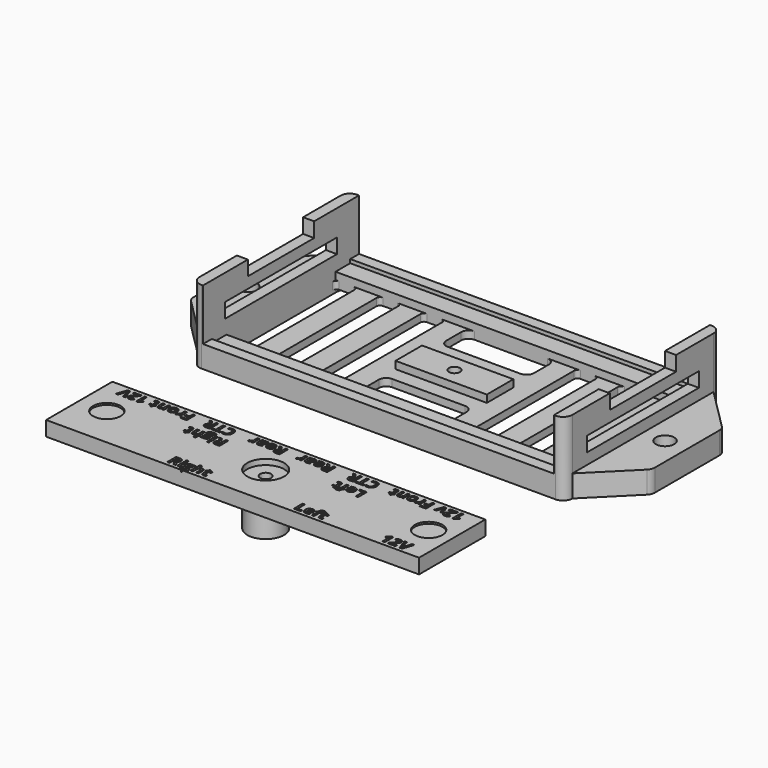
from build123d import *

# Parameters (mm, degrees)
F0_W            = 24.8000000916
F0_H            = 9
F0_W_2          = 95.3
F0_H_2          = 5
F0_R            = 2.5
F0_H_3          = 3
F0_W_3          = 47.65
F0_R_2          = 1.5
F1_DEPTH        = 3
F2_DEPTH        = 17
F3_DEPTH        = 2
F4_DEPTH        = 3
F5_W            = 3
F5_H            = 22.5
F6_W            = 3
F6_H            = 22.5
F7_DEPTH        = 4
F0_W_4          = 101.3
F0_H_4          = 22.5
F0_R_3          = 5
F8_DEPTH        = 4
F9_DEPTH        = 10
F10_DEPTH       = 3
F11_R           = 5
F11_R_2         = 1.5
F12_DEPTH       = 1.5
F13_R           = 6
F13_R_2         = 5
F14_DEPTH       = 1.5
F15_TEXT_SIZE   = 4.254734022
F15_TEXT_SIZE_2 = 4.1666666667
F15_TEXT_SIZE_3 = 4.0404040404
F15_W           = 0.6204427083
F15_H           = 2.2747395833
F15_R           = 3.75
F16_DEPTH       = 0.5
F17_R           = 1.5
F18_DEPTH       = 1
F19_W           = 96.2200004339
F19_H           = 17.4200004339
F19_R           = 7.9304002091
F20_DEPTH       = 2
F22_DEPTH       = 2
F24_W           = 38
F24_H           = 4
F23_W           = 38
F23_H           = 4
F25_DEPTH       = 5.5
F21_R           = 4.5
F21_R_2         = 1.5
F26_DEPTH       = 1


# Not quite as in the source:
# - a feature names something its author has since deleted; it is built from what else it names
# - Text() gives the source's letters only with a copy of the font that has no kerning and outlines rounded to 1/6400 em; it was checked with that copy


with BuildPart() as f1:
    # F0 (on Top) → F1 (new body)
    with BuildSketch(Plane.XY):
        Polygon((49.3014014482, 10.8854821861), (-45.9985985518, 10.8854821861), (-45.9985985518, -26.1145178139), (1.6514014482, -26.1145178139), (49.3014014482, -26.1145178139), align=None)
        with Locations((1.9014014941, -8.6145178139)):
            Rectangle(F0_W, F0_H, mode=Mode.SUBTRACT)
        with Locations((1.6514014482, 13.3854821861)):
            Rectangle(F0_W_2, F0_H_2)
        with BuildLine():
            Line((-48.9985985518, -31.5745178139), (-48.9985985518, 16.3454821861))
            Line((-48.9985985518, 16.3454821861), (-60.2531511942, 5.1096871314))
            ThreePointArc((-60.2531511942, 5.1096871314), (-60.804847016, 4.2851329962), (-60.9985985518, 3.3121385747))
            Line((-60.9985985518, 3.3121385747), (-60.9985985518, -18.5411742026))
            ThreePointArc((-60.9985985518, -18.5411742026), (-60.804847016, -19.514168624), (-60.2531511942, -20.3387227592))
            Line((-60.2531511942, -20.3387227592), (-48.9985985518, -31.5745178139))
        make_face()
        with Locations((-54.9985985518, -7.6145178139)):
            Circle(F0_R, mode=Mode.SUBTRACT)
        with BuildLine():
            Line((63.5559540907, 5.1096871314), (52.3014014482, 16.3454821861))
            Line((52.3014014482, 16.3454821861), (52.3014014482, -31.5745178139))
            Line((52.3014014482, -31.5745178139), (63.5559540907, -20.3387227592))
            ThreePointArc((63.5559540907, -20.3387227592), (64.1076499125, -19.514168624), (64.3014014482, -18.5411742026))
            Line((64.3014014482, -18.5411742026), (64.3014014482, -7.6145178139))
            Line((64.3014014482, -7.6145178139), (64.3014014482, 3.3121385747))
            ThreePointArc((64.3014014482, 3.3121385747), (64.1076499125, 4.2851329962), (63.5559540907, 5.1096871314))
        make_face()
        with Locations((58.3014014482, -7.6145178139)):
            Circle(F0_R, mode=Mode.SUBTRACT)
        with Locations((1.6514014482, 17.3854821861)):
            Rectangle(F0_W_2, F0_H_3)
        Polygon((1.6514014482, -31.1145178139), (-45.9985985518, -31.1145178139), (-45.9985985518, -34.1145178139), (49.3014014482, -34.1145178139), (49.3014014482, -31.1145178139), align=None)
        with Locations((-22.1735985518, -28.6145178139)):
            Rectangle(F0_W_3, F0_H_2)
        with Locations((25.4764014482, -28.6145178139)):
            Rectangle(F0_W_3, F0_H_2)
        with Locations((1.9014014941, -8.6145178139)):
            Rectangle(F0_W, F0_H)
        with Locations((1.9014014941, -8.6145178139)):
            Circle(F0_R_2, mode=Mode.SUBTRACT)
        with BuildLine():
            Line((49.3014014482, 18.8854821861), (49.3014014482, 15.8854821861))
            Line((49.3014014482, 15.8854821861), (49.3014014482, 10.8854821861))
            Line((49.3014014482, 10.8854821861), (49.3014014482, -26.1145178139))
            Line((49.3014014482, -26.1145178139), (49.3014014482, -31.1145178139))
            Line((49.3014014482, -31.1145178139), (49.3014014482, -34.1145178139))
            Line((49.3014014482, -34.1145178139), (49.7614014482, -34.1145178139))
            ThreePointArc((49.7614014482, -34.1145178139), (51.5574526725, -33.3705690381), (52.3014014482, -31.5745178139))
            Line((52.3014014482, -31.5745178139), (52.3014014482, 16.3454821861))
            ThreePointArc((52.3014014482, 16.3454821861), (51.5574526725, 18.1415334103), (49.7614014482, 18.8854821861))
            Line((49.7614014482, 18.8854821861), (49.3014014482, 18.8854821861))
        make_face()
        with BuildLine():
            Line((-45.9985985518, 10.8854821861), (-45.9985985518, 15.8854821861))
            Line((-45.9985985518, 15.8854821861), (-45.9985985518, 18.8854821861))
            Line((-45.9985985518, 18.8854821861), (-46.4585985518, 18.8854821861))
            ThreePointArc((-46.4585985518, 18.8854821861), (-48.254649776, 18.1415334103), (-48.9985985518, 16.3454821861))
            Line((-48.9985985518, 16.3454821861), (-48.9985985518, -31.5745178139))
            ThreePointArc((-48.9985985518, -31.5745178139), (-48.254649776, -33.3705690381), (-46.4585985518, -34.1145178139))
            Line((-46.4585985518, -34.1145178139), (-45.9985985518, -34.1145178139))
            Line((-45.9985985518, -34.1145178139), (-45.9985985518, -31.1145178139))
            Line((-45.9985985518, -31.1145178139), (-45.9985985518, -26.1145178139))
            Line((-45.9985985518, -26.1145178139), (-45.9985985518, 10.8854821861))
        make_face()
    extrude(amount=-F1_DEPTH)

    # F0 (on Top) → F2 (join)
    with BuildSketch(Plane.XY):
        with BuildLine():
            Line((49.3014014482, 18.8854821861), (49.3014014482, 15.8854821861))
            Line((49.3014014482, 15.8854821861), (49.3014014482, 10.8854821861))
            Line((49.3014014482, 10.8854821861), (49.3014014482, -26.1145178139))
            Line((49.3014014482, -26.1145178139), (49.3014014482, -31.1145178139))
            Line((49.3014014482, -31.1145178139), (49.3014014482, -34.1145178139))
            Line((49.3014014482, -34.1145178139), (49.7614014482, -34.1145178139))
            ThreePointArc((49.7614014482, -34.1145178139), (51.5574526725, -33.3705690381), (52.3014014482, -31.5745178139))
            Line((52.3014014482, -31.5745178139), (52.3014014482, 16.3454821861))
            ThreePointArc((52.3014014482, 16.3454821861), (51.5574526725, 18.1415334103), (49.7614014482, 18.8854821861))
            Line((49.7614014482, 18.8854821861), (49.3014014482, 18.8854821861))
        make_face()
        with BuildLine():
            Line((-45.9985985518, 10.8854821861), (-45.9985985518, 15.8854821861))
            Line((-45.9985985518, 15.8854821861), (-45.9985985518, 18.8854821861))
            Line((-45.9985985518, 18.8854821861), (-46.4585985518, 18.8854821861))
            ThreePointArc((-46.4585985518, 18.8854821861), (-48.254649776, 18.1415334103), (-48.9985985518, 16.3454821861))
            Line((-48.9985985518, 16.3454821861), (-48.9985985518, -31.5745178139))
            ThreePointArc((-48.9985985518, -31.5745178139), (-48.254649776, -33.3705690381), (-46.4585985518, -34.1145178139))
            Line((-46.4585985518, -34.1145178139), (-45.9985985518, -34.1145178139))
            Line((-45.9985985518, -34.1145178139), (-45.9985985518, -31.1145178139))
            Line((-45.9985985518, -31.1145178139), (-45.9985985518, -26.1145178139))
            Line((-45.9985985518, -26.1145178139), (-45.9985985518, 10.8854821861))
        make_face()
    extrude(amount=F2_DEPTH)

    # F0 (on Top) → F3 (join)
    with BuildSketch(Plane.XY):
        with Locations((1.9014014941, -8.6145178139)):
            Rectangle(F0_W, F0_H)
        with Locations((1.9014014941, -8.6145178139)):
            Circle(F0_R_2, mode=Mode.SUBTRACT)
        with Locations((1.6514014482, 13.3854821861)):
            Rectangle(F0_W_2, F0_H_2)
        with Locations((-22.1735985518, -28.6145178139)):
            Rectangle(F0_W_3, F0_H_2)
        with Locations((25.4764014482, -28.6145178139)):
            Rectangle(F0_W_3, F0_H_2)
    extrude(amount=F3_DEPTH)

    # F0 (on Top) → F4 (join)
    with BuildSketch(Plane.XY):
        with Locations((1.6514014482, 17.3854821861)):
            Rectangle(F0_W_2, F0_H_3)
        Polygon((1.6514014482, -31.1145178139), (-45.9985985518, -31.1145178139), (-45.9985985518, -34.1145178139), (49.3014014482, -34.1145178139), (49.3014014482, -31.1145178139), align=None)
    extrude(amount=F4_DEPTH)

    # F5 (on face) + F6 (on face) → F7 (cut)
    with BuildSketch(Plane.XY.offset(17)):
        with Locations((50.8014014482, -7.6145178139)):
            Rectangle(F5_W, F5_H)
    with BuildSketch(Plane.XY.offset(17)):
        with Locations((-47.4985985518, -7.6145178139)):
            Rectangle(F6_W, F6_H)
    extrude(amount=-F7_DEPTH, mode=Mode.SUBTRACT)

    # F0 (on Top) → F10 (join)
    with BuildSketch(Plane.XY):
        with BuildLine():
            Line((-48.9985985518, -31.5745178139), (-48.9985985518, 16.3454821861))
            Line((-48.9985985518, 16.3454821861), (-60.2531511942, 5.1096871314))
            ThreePointArc((-60.2531511942, 5.1096871314), (-60.804847016, 4.2851329962), (-60.9985985518, 3.3121385747))
            Line((-60.9985985518, 3.3121385747), (-60.9985985518, -18.5411742026))
            ThreePointArc((-60.9985985518, -18.5411742026), (-60.804847016, -19.514168624), (-60.2531511942, -20.3387227592))
            Line((-60.2531511942, -20.3387227592), (-48.9985985518, -31.5745178139))
        make_face()
        with Locations((-54.9985985518, -7.6145178139)):
            Circle(F0_R, mode=Mode.SUBTRACT)
        with BuildLine():
            Line((63.5559540907, 5.1096871314), (52.3014014482, 16.3454821861))
            Line((52.3014014482, 16.3454821861), (52.3014014482, -31.5745178139))
            Line((52.3014014482, -31.5745178139), (63.5559540907, -20.3387227592))
            ThreePointArc((63.5559540907, -20.3387227592), (64.1076499125, -19.514168624), (64.3014014482, -18.5411742026))
            Line((64.3014014482, -18.5411742026), (64.3014014482, -7.6145178139))
            Line((64.3014014482, -7.6145178139), (64.3014014482, 3.3121385747))
            ThreePointArc((64.3014014482, 3.3121385747), (64.1076499125, 4.2851329962), (63.5559540907, 5.1096871314))
        make_face()
        with Locations((58.3014014482, -7.6145178139)):
            Circle(F0_R, mode=Mode.SUBTRACT)
    extrude(amount=F10_DEPTH)

    # F17 (on face) → F18 (cut)
    with BuildSketch(Plane(origin=(0, 0, -3), x_dir=(1, 0, 0), z_dir=(0, 0, -1))):
        with BuildLine():
            ThreePointArc((-45.9985985518, -10.8854821861), (-44.5341324577, -14.421016092), (-40.9985985518, -15.8854821861))
            Line((-40.9985985518, -15.8854821861), (44.3014014482, -15.8854821861))
            ThreePointArc((44.3014014482, -15.8854821861), (47.8369353542, -14.421016092), (49.3014014482, -10.8854821861))
            Line((49.3014014482, -10.8854821861), (49.3014014482, 26.1145178139))
            ThreePointArc((49.3014014482, 26.1145178139), (47.8369353542, 29.6500517199), (44.3014014482, 31.1145178139))
            Line((44.3014014482, 31.1145178139), (-40.9985985518, 31.1145178139))
            ThreePointArc((-40.9985985518, 31.1145178139), (-44.5341324577, 29.6500517199), (-45.9985985518, 26.1145178139))
            Line((-45.9985985518, 26.1145178139), (-45.9985985518, -10.8854821861))
        make_face()
        with Locations((1.9014014941, 8.6145178139)):
            Circle(F17_R, mode=Mode.SUBTRACT)
    extrude(amount=-F18_DEPTH, mode=Mode.SUBTRACT)

    # F21 (on face) → F22 (cut)
    with BuildSketch(Plane(origin=(0, 0, -2), x_dir=(1, 0, 0), z_dir=(0, 0, -1))):
        with BuildLine():
            ThreePointArc((48.3014014482, -10.8854821861), (49.0085082294, -10.5925889673), (49.3014014482, -9.8854821861))
            Line((49.3014014482, -9.8854821861), (49.3014014482, 25.1145178139))
            ThreePointArc((49.3014014482, 25.1145178139), (49.0085082294, 25.8216245951), (48.3014014482, 26.1145178139))
            Line((48.3014014482, 26.1145178139), (44.3451514482, 26.1145178139))
            ThreePointArc((44.3451514482, 26.1145178139), (43.6380446671, 25.8216245951), (43.3451514482, 25.1145178139))
            Line((43.3451514482, 25.1145178139), (43.3451514482, -9.8854821861))
            ThreePointArc((43.3451514482, -9.8854821861), (43.6380446671, -10.5925889673), (44.3451514482, -10.8854821861))
            Line((44.3451514482, -10.8854821861), (48.3014014482, -10.8854821861))
        make_face()
        with BuildLine():
            Line((37.3889014482, -9.8854821861), (37.3889014482, 25.1145178139))
            ThreePointArc((37.3889014482, 25.1145178139), (37.0960082294, 25.8216245951), (36.3889014482, 26.1145178139))
            Line((36.3889014482, 26.1145178139), (32.4326514482, 26.1145178139))
            ThreePointArc((32.4326514482, 26.1145178139), (31.7255446671, 25.8216245951), (31.4326514482, 25.1145178139))
            Line((31.4326514482, 25.1145178139), (31.4326514482, -9.8854821861))
            ThreePointArc((31.4326514482, -9.8854821861), (31.7255446671, -10.5925889673), (32.4326514482, -10.8854821861))
            Line((32.4326514482, -10.8854821861), (36.3889014482, -10.8854821861))
            ThreePointArc((36.3889014482, -10.8854821861), (37.0960082294, -10.5925889673), (37.3889014482, -9.8854821861))
        make_face()
        with BuildLine():
            ThreePointArc((24.4764014482, -10.8854821861), (25.1835082294, -10.5925889673), (25.4764014482, -9.8854821861))
            Line((25.4764014482, -9.8854821861), (25.4764014482, 25.1145178139))
            ThreePointArc((25.4764014482, 25.1145178139), (25.1835082294, 25.8216245951), (24.4764014482, 26.1145178139))
            Line((24.4764014482, 26.1145178139), (20.5201514482, 26.1145178139))
            ThreePointArc((20.5201514482, 26.1145178139), (19.8130446671, 25.8216245951), (19.5201514482, 25.1145178139))
            Line((19.5201514482, 25.1145178139), (19.5201514482, -9.8854821861))
            ThreePointArc((19.5201514482, -9.8854821861), (19.8130446671, -10.5925889673), (20.5201514482, -10.8854821861))
            Line((20.5201514482, -10.8854821861), (24.4764014482, -10.8854821861))
        make_face()
        with BuildLine():
            Line((-22.1735985518, 25.1145178139), (-22.1735985518, -9.8854821861))
            ThreePointArc((-22.1735985518, -9.8854821861), (-21.8807053329, -10.5925889673), (-21.1735985518, -10.8854821861))
            Line((-21.1735985518, -10.8854821861), (-17.2173485518, -10.8854821861))
            ThreePointArc((-17.2173485518, -10.8854821861), (-16.5102417706, -10.5925889673), (-16.2173485518, -9.8854821861))
            Line((-16.2173485518, -9.8854821861), (-16.2173485518, 25.1145178139))
            ThreePointArc((-16.2173485518, 25.1145178139), (-16.5102417706, 25.8216245951), (-17.2173485518, 26.1145178139))
            Line((-17.2173485518, 26.1145178139), (-21.1735985518, 26.1145178139))
            ThreePointArc((-21.1735985518, 26.1145178139), (-21.8807053329, 25.8216245951), (-22.1735985518, 25.1145178139))
        make_face()
        with BuildLine():
            ThreePointArc((-33.0860985518, 26.1145178139), (-33.7932053329, 25.8216245951), (-34.0860985518, 25.1145178139))
            Line((-34.0860985518, 25.1145178139), (-34.0860985518, -9.8854821861))
            ThreePointArc((-34.0860985518, -9.8854821861), (-33.7932053329, -10.5925889673), (-33.0860985518, -10.8854821861))
            Line((-33.0860985518, -10.8854821861), (-29.1298485518, -10.8854821861))
            ThreePointArc((-29.1298485518, -10.8854821861), (-28.4227417706, -10.5925889673), (-28.1298485518, -9.8854821861))
            Line((-28.1298485518, -9.8854821861), (-28.1298485518, 25.1145178139))
            ThreePointArc((-28.1298485518, 25.1145178139), (-28.4227417706, 25.8216245951), (-29.1298485518, 26.1145178139))
            Line((-29.1298485518, 26.1145178139), (-33.0860985518, 26.1145178139))
        make_face()
        with BuildLine():
            ThreePointArc((-45.9985985518, -9.8854821861), (-45.7057053329, -10.5925889673), (-44.9985985518, -10.8854821861))
            Line((-44.9985985518, -10.8854821861), (-41.0423485518, -10.8854821861))
            ThreePointArc((-41.0423485518, -10.8854821861), (-40.3352417706, -10.5925889673), (-40.0423485518, -9.8854821861))
            Line((-40.0423485518, -9.8854821861), (-40.0423485518, 25.1145178139))
            ThreePointArc((-40.0423485518, 25.1145178139), (-40.3352417706, 25.8216245951), (-41.0423485518, 26.1145178139))
            Line((-41.0423485518, 26.1145178139), (-44.9985985518, 26.1145178139))
            ThreePointArc((-44.9985985518, 26.1145178139), (-45.7057053329, 25.8216245951), (-45.9985985518, 25.1145178139))
            Line((-45.9985985518, 25.1145178139), (-45.9985985518, -9.8854821861))
        make_face()
        with BuildLine():
            ThreePointArc((13.5639014482, 24.1145178139), (12.9781150106, 25.5287313763), (11.5639014482, 26.1145178139))
            Line((11.5639014482, 26.1145178139), (-8.2610985518, 26.1145178139))
            ThreePointArc((-8.2610985518, 26.1145178139), (-9.6753121141, 25.5287313763), (-10.2610985518, 24.1145178139))
            Line((-10.2610985518, 24.1145178139), (-10.2610985518, 19.0735178139))
            ThreePointArc((-10.2610985518, 19.0735178139), (-9.6753121141, 17.6593042515), (-8.2610985518, 17.0735178139))
            Line((-8.2610985518, 17.0735178139), (11.5639014482, 17.0735178139))
            ThreePointArc((11.5639014482, 17.0735178139), (12.9781150106, 17.6593042515), (13.5639014482, 19.0735178139))
            Line((13.5639014482, 19.0735178139), (13.5639014482, 24.1145178139))
        make_face()
        with BuildLine():
            Line((-8.2610985518, -10.8854821861), (11.5639014482, -10.8854821861))
            ThreePointArc((11.5639014482, -10.8854821861), (12.9781150106, -10.2996957485), (13.5639014482, -8.8854821861))
            Line((13.5639014482, -8.8854821861), (13.5639014482, -3.8114821861))
            ThreePointArc((13.5639014482, -3.8114821861), (12.9781150106, -2.3972686237), (11.5639014482, -1.8114821861))
            Line((11.5639014482, -1.8114821861), (-8.2610985518, -1.8114821861))
            ThreePointArc((-8.2610985518, -1.8114821861), (-9.6753121141, -2.3972686237), (-10.2610985518, -3.8114821861))
            Line((-10.2610985518, -3.8114821861), (-10.2610985518, -8.8854821861))
            ThreePointArc((-10.2610985518, -8.8854821861), (-9.6753121141, -10.2996957485), (-8.2610985518, -10.8854821861))
        make_face()
    extrude(amount=-F22_DEPTH, mode=Mode.SUBTRACT)

    # F24 (on face) + F23 (on face) → F25 (cut, symmetric)
    with BuildSketch(Plane(origin=(-48.9985985518, 0, 0), x_dir=(0, -1, 0), z_dir=(-1, 0, 0))):
        with Locations((7.6145178139, 8)):
            Rectangle(F24_W, F24_H)
    with BuildSketch(Plane.YZ.offset(52.3014014482)):
        with Locations((-7.6145178139, 8)):
            Rectangle(F23_W, F23_H)
    extrude(amount=F25_DEPTH, both=True, dir=(-1, 0, 0), mode=Mode.SUBTRACT)

    # F21 (on face) → F26 (join, through all)
    with BuildSketch(Plane(origin=(0, 0, -2), x_dir=(1, 0, 0), z_dir=(0, 0, -1))):
        with Locations((1.9014014941, 8.6145178139)):
            Circle(F21_R)
        with Locations((1.9014014941, 8.6145178139)):
            Circle(F21_R_2, mode=Mode.SUBTRACT)
    extrude(amount=F26_DEPTH)


with BuildPart() as f8:
    # F0 (on Top) → F8 (new body)
    with BuildSketch(Plane.XY):
        with Locations((1.6514019907, -72.3777604103)):
            Rectangle(F0_W_4, F0_H_4)
        with Locations((1.6514019907, -72.3777604103)):
            Circle(F0_R_3, mode=Mode.SUBTRACT)
        with Locations((1.6514019907, -72.3777604103)):
            Circle(F0_R_3)
        with Locations((1.6514019907, -72.3777604103)):
            Circle(F0_R_2, mode=Mode.SUBTRACT)
    extrude(amount=F8_DEPTH)

    # F0 (on Top) → F9 (join)
    with BuildSketch(Plane.XY):
        with Locations((1.6514019907, -72.3777604103)):
            Circle(F0_R_3)
        with Locations((1.6514019907, -72.3777604103)):
            Circle(F0_R_2, mode=Mode.SUBTRACT)
    extrude(amount=-F9_DEPTH)

    # F11 (on face) → F12 (cut)
    with BuildSketch(Plane.XY.offset(4)):
        with Locations((1.6514019907, -72.3777604103)):
            Circle(F11_R)
        with Locations((1.6514019907, -72.3777604103)):
            Circle(F11_R_2, mode=Mode.SUBTRACT)
    extrude(amount=-F12_DEPTH, mode=Mode.SUBTRACT)

    # F13 (on face) → F14 (join)
    with BuildSketch(Plane.XY):
        with Locations((1.6514019907, -72.3777604103)):
            Circle(F13_R)
        with Locations((1.6514019907, -72.3777604103)):
            Circle(F13_R_2, mode=Mode.SUBTRACT)
    extrude(amount=-F14_DEPTH)

    # F15 (on face) → F16 (cut)
    with BuildSketch(Plane.XY.offset(4)):
        with Locations(Location((48.2781432374, -62.1277615428), (0, 0, 180))):
            Text('12v', F15_TEXT_SIZE, font='Open Sans', font_style=FontStyle.BOLD, text_align=(TextAlign.LEFT, TextAlign.BOTTOM))
        with Locations(Location((39.7224306365, -62.1277615428), (0, 0, 180))):
            Text('Front', F15_TEXT_SIZE_2, font='Open Sans', font_style=FontStyle.BOLD, text_align=(TextAlign.LEFT, TextAlign.BOTTOM))
        with Locations(Location((25.045672824, -62.1277615428), (0, 0, 180))):
            Text('CTR', F15_TEXT_SIZE_2, font='Open Sans', font_style=FontStyle.BOLD, text_align=(TextAlign.LEFT, TextAlign.BOTTOM))
        with Locations(Location((25.188250949, -67.0007616282), (0, 0, 180))):
            Text('Left', F15_TEXT_SIZE_2, font='Open Sans', font_style=FontStyle.BOLD, text_align=(TextAlign.LEFT, TextAlign.BOTTOM))
        with Locations(Location((12.9034202198, -62.1277638078), (0, 0, 180))):
            Text('Rear', F15_TEXT_SIZE_2, font='Open Sans', font_style=FontStyle.BOLD, text_align=(TextAlign.LEFT, TextAlign.BOTTOM))
        with Locations(Location((-0.0965797802, -62.1277615428), (0, 0, 180))):
            Text('Rear', F15_TEXT_SIZE_2, font='Open Sans', font_style=FontStyle.BOLD, text_align=(TextAlign.LEFT, TextAlign.BOTTOM))
        with Locations(Location((-13.954327176, -62.1277615428), (0, 0, 180))):
            Text('CTR', F15_TEXT_SIZE_2, font='Open Sans', font_style=FontStyle.BOLD, text_align=(TextAlign.LEFT, TextAlign.BOTTOM))
        with Locations(Location((-12.4689761202, -67.0007615428), (0, 0, 180))):
            Text('Right', F15_TEXT_SIZE_2, font='Open Sans', font_style=FontStyle.BOLD, text_align=(TextAlign.LEFT, TextAlign.BOTTOM))
        with Locations(Location((-25.2775693635, -62.1277615428), (0, 0, 180))):
            Text('Front', F15_TEXT_SIZE_2, font='Open Sans', font_style=FontStyle.BOLD, text_align=(TextAlign.LEFT, TextAlign.BOTTOM))
        with Locations(Location((-37.7485980093, -62.1580645731), (0, 0, 180))):
            Text('12V', F15_TEXT_SIZE_3, font='Open Sans', font_style=FontStyle.BOLD, text_align=(TextAlign.LEFT, TextAlign.BOTTOM))
        with BuildLine():
            Line((-16.2230120718, -82.6277583838), (-16.2230120718, -81.4864823421))
            Line((-16.2230120718, -81.4864823421), (-15.8877256135, -81.4864823421))
            Line((-15.8877256135, -81.4864823421), (-15.1774391552, -82.6277583838))
            Line((-15.1774391552, -82.6277583838), (-14.4775693635, -82.6277583838))
            add(Edge.make_bspline(
                [(-15.3525693635, -81.3315344254), (-14.6806943635, -82.3347896338), (-14.4775693635, -82.6277583838)],
                knots=[0, 0, 0, 1, 1, 1], degree=2))
            add(Edge.make_bspline(
                [(-14.943389676, -81.0112219254), (-15.0875954052, -81.2156490088), (-15.3525693635, -81.3315344254)],
                knots=[0, 0, 0, 1, 1, 1], degree=2))
            add(Edge.make_bspline(
                [(-14.7991839468, -80.5444250504), (-14.7991839468, -80.8067948421), (-14.943389676, -81.0112219254)],
                knots=[0, 0, 0, 1, 1, 1], degree=2))
            add(Edge.make_bspline(
                [(-15.089874051, -79.8738521338), (-14.7991839468, -80.0945552588), (-14.7991839468, -80.5444250504)],
                knots=[0, 0, 0, 1, 1, 1], degree=2))
            add(Edge.make_bspline(
                [(-15.9873349885, -79.6531490088), (-15.3805641552, -79.6531490088), (-15.089874051, -79.8738521338)],
                knots=[0, 0, 0, 1, 1, 1], degree=2))
            Line((-15.9873349885, -79.6531490088), (-16.8538714468, -79.6531490088))
            Line((-16.8538714468, -79.6531490088), (-16.8538714468, -82.6277583838))
            Line((-16.8538714468, -82.6277583838), (-16.2230120718, -82.6277583838))
        make_face()
        with BuildLine():
            Line((-16.0198870718, -80.9734615088), (-16.2230120718, -80.9734615088))
            Line((-16.2230120718, -80.9734615088), (-16.2230120718, -80.1700760921))
            Line((-16.2230120718, -80.1700760921), (-16.0316058218, -80.1700760921))
            add(Edge.make_bspline(
                [(-15.5814105093, -80.2595943213), (-15.7269183218, -80.1700760921), (-16.0316058218, -80.1700760921)],
                knots=[0, 0, 0, 1, 1, 1], degree=2))
            add(Edge.make_bspline(
                [(-15.4359026968, -80.5607010921), (-15.4359026968, -80.3491125504), (-15.5814105093, -80.2595943213)],
                knots=[0, 0, 0, 1, 1, 1], degree=2))
            add(Edge.make_bspline(
                [(-15.578155301, -80.8738521338), (-15.4359026968, -80.7742427588), (-15.4359026968, -80.5607010921)],
                knots=[0, 0, 0, 1, 1, 1], degree=2))
            add(Edge.make_bspline(
                [(-16.0198870718, -80.9734615088), (-15.7204079052, -80.9734615088), (-15.578155301, -80.8738521338)],
                knots=[0, 0, 0, 1, 1, 1], degree=2))
        make_face(mode=Mode.SUBTRACT)
        with BuildLine():
            add(Edge.make_bspline(
                [(-14.1787412385, -79.7651281754), (-14.1787412385, -79.4617427588), (-13.8408506135, -79.4617427588)],
                knots=[0, 0, 0, 1, 1, 1], degree=2))
            add(Edge.make_bspline(
                [(-13.8408506135, -80.0704667171), (-14.1787412385, -80.0704667171), (-14.1787412385, -79.7651281754)],
                knots=[0, 0, 0, 1, 1, 1], degree=2))
            add(Edge.make_bspline(
                [(-13.5872698843, -79.9900630713), (-13.6715797802, -80.0704667171), (-13.8408506135, -80.0704667171)],
                knots=[0, 0, 0, 1, 1, 1], degree=2))
            add(Edge.make_bspline(
                [(-13.5029599885, -79.7651281754), (-13.5029599885, -79.9096594254), (-13.5872698843, -79.9900630713)],
                knots=[0, 0, 0, 1, 1, 1], degree=2))
            add(Edge.make_bspline(
                [(-13.8408506135, -79.4617427588), (-13.5029599885, -79.4617427588), (-13.5029599885, -79.7651281754)],
                knots=[0, 0, 0, 1, 1, 1], degree=2))
        make_face()
        with Locations((-13.841827176, -81.4903885921)):
            Rectangle(F15_W, F15_H)
        with BuildLine():
            add(Edge.make_bspline(
                [(-12.2976699022, -83.6277604103), (-12.7133493907, -83.6143693222), (-12.9424131135, -83.4630448421)],
                knots=[0.0884925433, 0.0884925433, 0.0884925433, 1, 1, 1], degree=2))
            Line((-12.2976699022, -83.6277604103), (-12.1211642128, -83.6277604103))
            add(Edge.make_bspline(
                [(-11.6985980093, -83.5814627277), (-11.8880167396, -83.6211940979), (-12.1211642128, -83.6277604103)],
                knots=[0.5345726688, 0.5345726688, 0.5345726688, 0.9230798932, 0.9230798932, 0.9230798932], degree=2))
            add(Edge.make_bspline(
                [(-11.2601214468, -83.4093339046), (-11.4379643074, -83.5267937195), (-11.6985980093, -83.5814627277)],
                knots=[0, 0, 0, 0.5345726688, 0.5345726688, 0.5345726688], degree=2))
            add(Edge.make_bspline(
                [(-10.9274391552, -82.7905188004), (-10.9274391552, -83.1896073421), (-11.2601214468, -83.4093339046)],
                knots=[0, 0, 0, 1, 1, 1], degree=2))
            add(Edge.make_bspline(
                [(-11.1237282177, -82.3185135921), (-10.9274391552, -82.4793208838), (-10.9274391552, -82.7905188004)],
                knots=[0, 0, 0, 1, 1, 1], degree=2))
            add(Edge.make_bspline(
                [(-11.6943662385, -82.1577063004), (-11.3200172802, -82.1577063004), (-11.1237282177, -82.3185135921)],
                knots=[0, 0, 0, 1, 1, 1], degree=2))
            Line((-11.6943662385, -82.1577063004), (-12.0810849885, -82.1577063004))
            add(Edge.make_bspline(
                [(-12.4228818635, -82.0235917171), (-12.4228818635, -82.1577063004), (-12.0810849885, -82.1577063004)],
                knots=[0, 0, 0, 1, 1, 1], degree=2))
            add(Edge.make_bspline(
                [(-12.3271787385, -81.8608313004), (-12.4228818635, -81.9337479671), (-12.4228818635, -82.0235917171)],
                knots=[0, 0, 0, 1, 1, 1], degree=2))
            Line((-12.3271787385, -81.8608313004), (-12.2353818635, -81.8705969254))
            Line((-12.2353818635, -81.8705969254), (-12.1234026968, -81.8771073421))
            add(Edge.make_bspline(
                [(-11.4147438427, -81.6726802588), (-11.6702776968, -81.8771073421), (-12.1234026968, -81.8771073421)],
                knots=[0, 0, 0, 1, 1, 1], degree=2))
            add(Edge.make_bspline(
                [(-11.1592099885, -81.1017167171), (-11.1592099885, -81.4682531754), (-11.4147438427, -81.6726802588)],
                knots=[0, 0, 0, 1, 1, 1], degree=2))
            add(Edge.make_bspline(
                [(-11.2568662385, -80.7599198421), (-11.1592099885, -80.9129146338), (-11.1592099885, -81.1017167171)],
                knots=[0, 0, 0, 1, 1, 1], degree=2))
            Line((-11.2568662385, -80.7599198421), (-10.9007464468, -80.6687740088))
            Line((-10.9007464468, -80.6687740088), (-10.9007464468, -80.3530188004))
            Line((-10.9007464468, -80.3530188004), (-11.6943662385, -80.3530188004))
            add(Edge.make_bspline(
                [(-11.8620094677, -80.3279536963), (-11.7308245718, -80.3452063004), (-11.6943662385, -80.3530188004)],
                knots=[0, 0, 0, 1, 1, 1], degree=2))
            add(Edge.make_bspline(
                [(-12.0888974885, -80.3107010921), (-11.9931943635, -80.3107010921), (-11.8620094677, -80.3279536963)],
                knots=[0, 0, 0, 1, 1, 1], degree=2))
            add(Edge.make_bspline(
                [(-12.7809547802, -80.5141516129), (-12.5387672802, -80.3107010921), (-12.0888974885, -80.3107010921)],
                knots=[0, 0, 0, 1, 1, 1], degree=2))
            add(Edge.make_bspline(
                [(-13.0231422802, -81.0893469254), (-13.0231422802, -80.7176021338), (-12.7809547802, -80.5141516129)],
                knots=[0, 0, 0, 1, 1, 1], degree=2))
            add(Edge.make_bspline(
                [(-12.9183245718, -81.4926672379), (-13.0231422802, -81.3217688004), (-13.0231422802, -81.0893469254)],
                knots=[0, 0, 0, 1, 1, 1], degree=2))
            add(Edge.make_bspline(
                [(-12.6344704052, -81.7403885921), (-12.8135068635, -81.6635656754), (-12.9183245718, -81.4926672379)],
                knots=[0, 0, 0, 1, 1, 1], degree=2))
            add(Edge.make_bspline(
                [(-12.8522438427, -81.9106359879), (-12.7770485302, -81.8243729671), (-12.6344704052, -81.7403885921)],
                knots=[0, 0, 0, 1, 1, 1], degree=2))
            add(Edge.make_bspline(
                [(-12.9274391552, -82.1271073421), (-12.9274391552, -81.9968990088), (-12.8522438427, -81.9106359879)],
                knots=[0, 0, 0, 1, 1, 1], degree=2))
            add(Edge.make_bspline(
                [(-12.8561500927, -82.3237219254), (-12.9274391552, -82.2312740088), (-12.9274391552, -82.1271073421)],
                knots=[0, 0, 0, 1, 1, 1], degree=2))
            add(Edge.make_bspline(
                [(-12.6891579052, -82.4565344254), (-12.7848610302, -82.4161698421), (-12.8561500927, -82.3237219254)],
                knots=[0, 0, 0, 1, 1, 1], degree=2))
            add(Edge.make_bspline(
                [(-13.0654599885, -82.6541255713), (-12.9372047802, -82.5157792171), (-12.6891579052, -82.4565344254)],
                knots=[0, 0, 0, 1, 1, 1], degree=2))
            add(Edge.make_bspline(
                [(-13.1937151968, -82.9982010921), (-13.1937151968, -82.7924719254), (-13.0654599885, -82.6541255713)],
                knots=[0, 0, 0, 1, 1, 1], degree=2))
            add(Edge.make_bspline(
                [(-12.9424131135, -83.4630448421), (-13.1937151968, -83.2970292171), (-13.1937151968, -82.9982010921)],
                knots=[0, 0, 0, 1, 1, 1], degree=2))
        make_face()
        with BuildLine():
            add(Edge.make_bspline(
                [(-11.6985980093, -83.1469899694), (-11.6818203751, -83.1399721206), (-11.666045926, -83.1323156754)],
                knots=[0.9165936185, 0.9165936185, 0.9165936185, 1, 1, 1], degree=2))
            add(Edge.make_bspline(
                [(-12.1885068635, -83.2241125504), (-11.8829756574, -83.2241125504), (-11.6985980093, -83.1469899694)],
                knots=[0, 0, 0, 0.9165936185, 0.9165936185, 0.9165936185], degree=2))
            add(Edge.make_bspline(
                [(-12.5335589468, -83.1508703629), (-12.4105120718, -83.2241125504), (-12.1885068635, -83.2241125504)],
                knots=[0, 0, 0, 1, 1, 1], degree=2))
            add(Edge.make_bspline(
                [(-12.6566058218, -82.9493729671), (-12.6566058218, -83.0776281754), (-12.5335589468, -83.1508703629)],
                knots=[0, 0, 0, 1, 1, 1], degree=2))
            add(Edge.make_bspline(
                [(-12.5416969677, -82.7368078629), (-12.6566058218, -82.8172115088), (-12.6566058218, -82.9493729671)],
                knots=[0, 0, 0, 1, 1, 1], degree=2))
            add(Edge.make_bspline(
                [(-12.2562151968, -82.6564042171), (-12.4267881135, -82.6564042171), (-12.5416969677, -82.7368078629)],
                knots=[0, 0, 0, 1, 1, 1], degree=2))
            Line((-12.2562151968, -82.6564042171), (-11.9346006135, -82.6564042171))
            add(Edge.make_bspline(
                [(-11.6985980093, -82.6737885249), (-11.7947530313, -82.6564042171), (-11.9346006135, -82.6564042171)],
                knots=[0.4033169827, 0.4033169827, 0.4033169827, 1, 1, 1], degree=2))
            add(Edge.make_bspline(
                [(-11.5885719677, -82.7052323421), (-11.6336037792, -82.68553913), (-11.6985980093, -82.6737885249)],
                knots=[0, 0, 0, 0.4033169827, 0.4033169827, 0.4033169827], degree=2))
            add(Edge.make_bspline(
                [(-11.4769183218, -82.8823156754), (-11.4769183218, -82.7540604671), (-11.5885719677, -82.7052323421)],
                knots=[0, 0, 0, 1, 1, 1], degree=2))
            add(Edge.make_bspline(
                [(-11.666045926, -83.1323156754), (-11.4769183218, -83.0405188004), (-11.4769183218, -82.8823156754)],
                knots=[0, 0, 0, 1, 1, 1], degree=2))
        make_face(mode=Mode.SUBTRACT)
        with BuildLine():
            add(Edge.make_bspline(
                [(-12.4306943635, -81.0978104671), (-12.4306943635, -81.2827063004), (-12.3463844677, -81.3907792171)],
                knots=[0, 0, 0, 1, 1, 1], degree=2))
            add(Edge.make_bspline(
                [(-12.0888974885, -80.6870031754), (-12.4306943635, -80.6870031754), (-12.4306943635, -81.0978104671)],
                knots=[0, 0, 0, 1, 1, 1], degree=2))
            add(Edge.make_bspline(
                [(-11.7516579052, -81.0978104671), (-11.7516579052, -80.6870031754), (-12.0888974885, -80.6870031754)],
                knots=[0, 0, 0, 1, 1, 1], degree=2))
            add(Edge.make_bspline(
                [(-11.8330381135, -81.3907792171), (-11.7516579052, -81.2827063004), (-11.7516579052, -81.0978104671)],
                knots=[0, 0, 0, 1, 1, 1], degree=2))
            add(Edge.make_bspline(
                [(-12.0888974885, -81.4988521338), (-11.9144183218, -81.4988521338), (-11.8330381135, -81.3907792171)],
                knots=[0, 0, 0, 1, 1, 1], degree=2))
            add(Edge.make_bspline(
                [(-12.3463844677, -81.3907792171), (-12.2620745718, -81.4988521338), (-12.0888974885, -81.4988521338)],
                knots=[0, 0, 0, 1, 1, 1], degree=2))
        make_face(mode=Mode.SUBTRACT)
        with BuildLine():
            Line((-9.0472308218, -82.6277583838), (-8.4267881135, -82.6277583838))
            Line((-8.4267881135, -82.6277583838), (-8.4267881135, -81.1446854671))
            add(Edge.make_bspline(
                [(-8.6341448843, -80.5261958838), (-8.4267881135, -80.7416906754), (-8.4267881135, -81.1446854671)],
                knots=[0, 0, 0, 1, 1, 1], degree=2))
            add(Edge.make_bspline(
                [(-9.2425433218, -80.3107010921), (-8.8415016552, -80.3107010921), (-8.6341448843, -80.5261958838)],
                knots=[0, 0, 0, 1, 1, 1], degree=2))
            add(Edge.make_bspline(
                [(-9.9020485302, -80.6440344254), (-9.6943662385, -80.3107010921), (-9.2425433218, -80.3107010921)],
                knots=[0, 0, 0, 1, 1, 1], degree=2))
            Line((-9.9020485302, -80.6440344254), (-9.9346006135, -80.6440344254))
            Line((-9.9346006135, -80.6440344254), (-9.9202776968, -80.4610917171))
            add(Edge.make_bspline(
                [(-9.9059547802, -80.1069250504), (-9.9059547802, -80.1824458838), (-9.9202776968, -80.4610917171)],
                knots=[0, 0, 0, 1, 1, 1], degree=2))
            Line((-9.9059547802, -80.1069250504), (-9.9059547802, -79.4617427588))
            Line((-9.9059547802, -79.4617427588), (-10.5263974885, -79.4617427588))
            Line((-10.5263974885, -79.4617427588), (-10.5263974885, -82.6277583838))
            Line((-10.5263974885, -82.6277583838), (-9.9059547802, -82.6277583838))
            Line((-9.9059547802, -82.6277583838), (-9.9059547802, -81.5574458838))
            add(Edge.make_bspline(
                [(-9.7900693635, -80.9838781754), (-9.9059547802, -81.1609615088), (-9.9059547802, -81.5574458838)],
                knots=[0, 0, 0, 1, 1, 1], degree=2))
            add(Edge.make_bspline(
                [(-9.4137672802, -80.8067948421), (-9.6741839468, -80.8067948421), (-9.7900693635, -80.9838781754)],
                knots=[0, 0, 0, 1, 1, 1], degree=2))
            add(Edge.make_bspline(
                [(-9.0472308218, -81.2989823421), (-9.0472308218, -80.8067948421), (-9.4137672802, -80.8067948421)],
                knots=[0, 0, 0, 1, 1, 1], degree=2))
            Line((-9.0472308218, -81.2989823421), (-9.0472308218, -82.6277583838))
        make_face()
        with BuildLine():
            add(Edge.make_bspline(
                [(-6.8297829052, -82.1739823421), (-6.6670224885, -82.1739823421), (-6.4391579052, -82.1030188004)],
                knots=[0, 0, 0, 1, 1, 1], degree=2))
            add(Edge.make_bspline(
                [(-7.0263974885, -82.1108313004), (-6.9521787385, -82.1739823421), (-6.8297829052, -82.1739823421)],
                knots=[0, 0, 0, 1, 1, 1], degree=2))
            add(Edge.make_bspline(
                [(-7.1006162385, -81.9155188004), (-7.1006162385, -82.0476802588), (-7.0263974885, -82.1108313004)],
                knots=[0, 0, 0, 1, 1, 1], degree=2))
            Line((-7.1006162385, -81.9155188004), (-7.1006162385, -80.8191646338))
            Line((-7.1006162385, -80.8191646338), (-6.4638974885, -80.8191646338))
            Line((-6.4638974885, -80.8191646338), (-6.4638974885, -80.3530188004))
            Line((-6.4638974885, -80.3530188004), (-7.1006162385, -80.3530188004))
            Line((-7.1006162385, -80.3530188004), (-7.1006162385, -79.8686438004))
            Line((-7.1006162385, -79.8686438004), (-7.4971006135, -79.8686438004))
            Line((-7.4971006135, -79.8686438004), (-7.6761370718, -80.3491125504))
            Line((-7.6761370718, -80.3491125504), (-8.0179339468, -80.5567948421))
            Line((-8.0179339468, -80.5567948421), (-8.0179339468, -80.8191646338))
            Line((-8.0179339468, -80.8191646338), (-7.7210589468, -80.8191646338))
            Line((-7.7210589468, -80.8191646338), (-7.7210589468, -81.9155188004))
            add(Edge.make_bspline(
                [(-7.5511370718, -82.4802974463), (-7.7210589468, -82.2918208838), (-7.7210589468, -81.9155188004)],
                knots=[0, 0, 0, 1, 1, 1], degree=2))
            add(Edge.make_bspline(
                [(-7.0088193635, -82.6687740088), (-7.3812151968, -82.6687740088), (-7.5511370718, -82.4802974463)],
                knots=[0, 0, 0, 1, 1, 1], degree=2))
            add(Edge.make_bspline(
                [(-6.4391579052, -82.5646073421), (-6.6709287385, -82.6687740088), (-7.0088193635, -82.6687740088)],
                knots=[0, 0, 0, 1, 1, 1], degree=2))
            Line((-6.4391579052, -82.5646073421), (-6.4391579052, -82.1030188004))
        make_face()
        with Locations((17.1145530323, -82.6277583838)):
            Text('Left', F15_TEXT_SIZE_2, font='Open Sans', font_style=FontStyle.BOLD, text_align=(TextAlign.LEFT, TextAlign.BOTTOM))
        with Locations((40.4342144907, -82.6277583838)):
            Text('12V', F15_TEXT_SIZE_2, font='Open Sans', font_style=FontStyle.BOLD, text_align=(TextAlign.LEFT, TextAlign.BOTTOM))
        with BuildLine():
            ThreePointArc((-37.7485980093, -72.3777604103), (-41.4985980093, -68.6277604103), (-45.2485980093, -72.3777604103))
            ThreePointArc((-45.2485980093, -72.3777604103), (-41.4985980093, -76.1277604103), (-37.7485980093, -72.3777604103))
        make_face()
        with Locations((45.9099337459, -72.3777604103)):
            Circle(F15_R)
    extrude(amount=-F16_DEPTH, mode=Mode.SUBTRACT)

    # F19 (on face) → F20 (cut)
    with BuildSketch(Plane.XY):
        with Locations((1.6514019907, -72.3777604103)):
            Rectangle(F19_W, F19_H)
        with Locations((1.6514019907, -72.3777604103)):
            Circle(F19_R, mode=Mode.SUBTRACT)
    extrude(amount=F20_DEPTH, mode=Mode.SUBTRACT)


solid = Compound([f1.part, f8.part])
